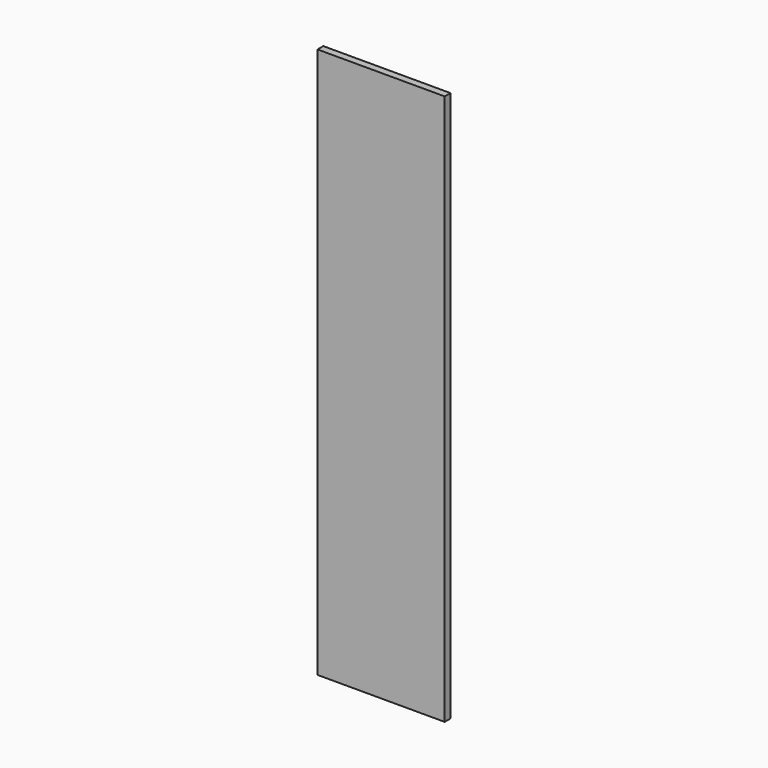
from build123d import *

# Parameters (mm, degrees)
F0_W     = 279.4
F0_H     = 1209.675
F1_DEPTH = 15.875


# Not quite as in the source:
# - a length typed as a fraction of an inch, garbled in the dataset ("3 / 203.2 mm" for 3/8 in), is restored


with BuildPart() as f1:
    # F0 (on Front) → F1 (new body)
    with BuildSketch(Plane.XZ):
        with Locations((139.7, 604.8375)):
            Rectangle(F0_W, F0_H)
    extrude(amount=F1_DEPTH)


solid = f1.part
